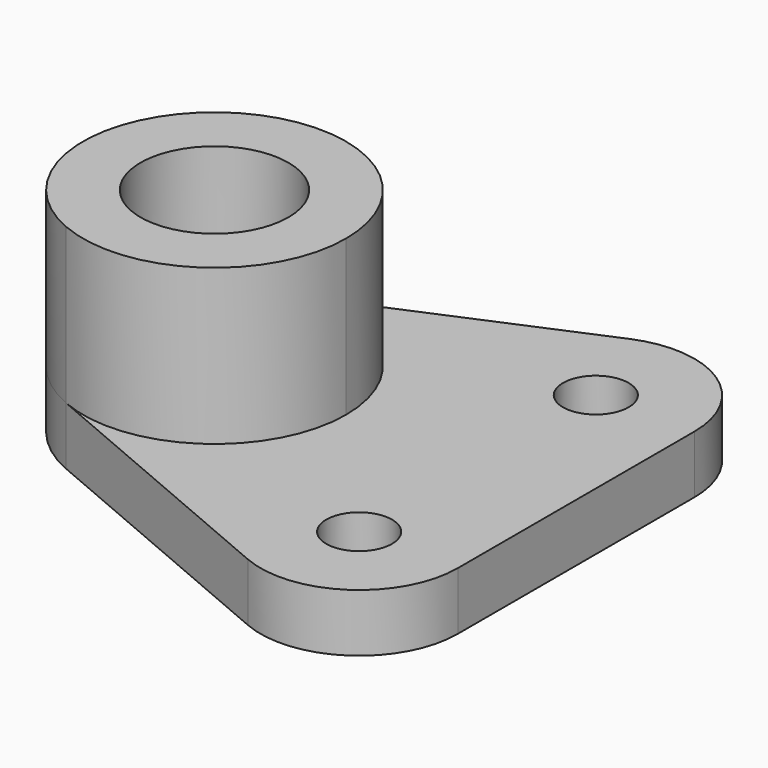
from build123d import *
from build123d import SkipClean  # not in build123d's __all__

# Parameters (mm, degrees)
F0_R     = 14.2875
F0_R_2   = 6.35
F1_DEPTH = 11.176
F2_DEPTH = 41.148
F3_DEPTH = 11.177
F4_DEPTH = 41.149


with BuildPart() as f1:
    # F0 (on Top) → F1 (new body)
    with BuildSketch(Plane.XY):
        with BuildLine():
            ThreePointArc((-61.399120046, 23.3629201096), (-37.4323475039, 21.1933093342), (-26.0324774843, 0))
            ThreePointArc((-26.0324774843, 0), (-37.4323475039, -21.1933093342), (-61.399120046, -23.3629201096))
            Line((-61.399120046, -23.3629201096), (-8.1074594056, -46.0971900822))
            ThreePointArc((-8.1074594056, -46.0971900822), (-11.1325749696, -12.6800179994), (18.4175225157, -28.575))
            Line((18.4175225157, -28.575), (18.4175225157, 28.575))
            ThreePointArc((18.4175225157, 28.575), (-11.1325749696, 12.6800179994), (-8.1074594056, 46.0971900822))
            Line((-8.1074594056, 46.0971900822), (-61.399120046, 23.3629201096))
        make_face()
        with BuildLine():
            ThreePointArc((-61.399120046, -23.3629201096), (-37.4323475039, -21.1933093342), (-26.0324774843, 0))
            ThreePointArc((-26.0324774843, 0), (-37.4323475039, 21.1933093342), (-61.399120046, 23.3629201096))
            ThreePointArc((-61.399120046, 23.3629201096), (-76.8324774843, 0), (-61.399120046, -23.3629201096))
        make_face()
        with Locations((-51.4324774843, 0)):
            Circle(F0_R, mode=Mode.SUBTRACT)
        with BuildLine():
            ThreePointArc((18.4175225157, 28.575), (9.867620001, 44.4699820006), (-8.1074594056, 46.0971900822))
            ThreePointArc((-8.1074594056, 46.0971900822), (-11.1325749696, 12.6800179994), (18.4175225157, 28.575))
        make_face()
        with Locations((-0.6324774843, 28.575)):
            Circle(F0_R_2, mode=Mode.SUBTRACT)
        with BuildLine():
            ThreePointArc((18.4175225157, -28.575), (-11.1325749696, -12.6800179994), (-8.1074594056, -46.0971900822))
            ThreePointArc((-8.1074594056, -46.0971900822), (9.867620001, -44.4699820006), (18.4175225157, -28.575))
        make_face()
        with Locations((-0.6324774843, -28.575)):
            Circle(F0_R_2, mode=Mode.SUBTRACT)
        with Locations((-51.4324774843, 0)):
            Circle(F0_R)
        with Locations((-0.6324774843, -28.575)):
            Circle(F0_R_2)
        with Locations((-0.6324774843, 28.575)):
            Circle(F0_R_2)
    extrude(amount=F1_DEPTH)

    # F0 (on Top) → F2 (join)
    with BuildSketch(Plane.XY):
        with BuildLine():
            ThreePointArc((-61.399120046, -23.3629201096), (-37.4323475039, -21.1933093342), (-26.0324774843, 0))
            ThreePointArc((-26.0324774843, 0), (-37.4323475039, 21.1933093342), (-61.399120046, 23.3629201096))
            ThreePointArc((-61.399120046, 23.3629201096), (-76.8324774843, 0), (-61.399120046, -23.3629201096))
        make_face()
        with Locations((-51.4324774843, 0)):
            Circle(F0_R, mode=Mode.SUBTRACT)
    with SkipClean():  # cleaning this boolean's faces spoils the solid; the shape is the same uncleaned
        extrude(amount=F2_DEPTH)

    # F3 (cut, through all): a face of the model
    f3_faces = [f1.faces().sort_by_distance(p)[0] for p in [
        (-51.4324774843, 0, 11.176),
    ]]
    with SkipClean():  # cleaning this boolean's faces spoils the solid; the shape is the same uncleaned
        extrude(f3_faces, amount=-F3_DEPTH, mode=Mode.SUBTRACT)

    # F0 (on Top) → F4 (cut, through all)
    with BuildSketch(Plane.XY):
        with Locations((-0.6324774843, 28.575)):
            Circle(F0_R_2)
        with Locations((-0.6324774843, -28.575)):
            Circle(F0_R_2)
    with SkipClean():  # cleaning this boolean's faces spoils the solid; the shape is the same uncleaned
        extrude(amount=F4_DEPTH, mode=Mode.SUBTRACT)


solid = f1.part
